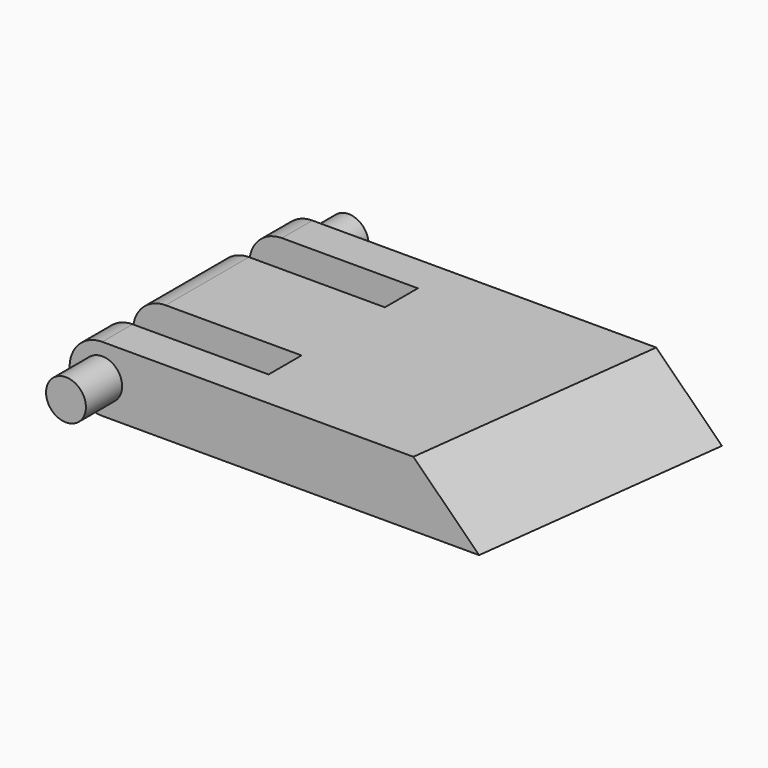
from build123d import *

# Parameters (mm, degrees)
F1_DEPTH  = 3.6
F2_SIZE2  = 3.59999
F2_SIZE   = 3.59999
F3_R      = 1.8
F4_R      = 1.79999
F5_R      = 1.8
F6_R      = 1.79999
F7_R      = 1.8
F8_R      = 1.79999
F9_R      = 1.1
F10_DEPTH = 2.5
F11_R     = 1.1
F12_DEPTH = 2.5


# Not quite as in the source:
# - a fillet or chamfer is up to 0.001 mm smaller than in the source, because OpenCascade refuses the exact size


with BuildPart() as f1:
    # F0 (on Top) → F1 (new body)
    with BuildSketch(Plane.XY):
        Polygon((24.4, 0), (0, 0), (0, -2.1), (9.3, -2.1), (9.3, -4.375), (0, -4.375), (0, -10.125), (9.3, -10.125), (9.3, -12.4), (0, -12.4), (0, -14.5), (22.6, -14.5), align=None)
    extrude(amount=F1_DEPTH)

    # F2 (size 3.6 and 3.6 in the source; OpenCascade refuses exactly that, so slightly less here)
    f2_edges = [f1.edges().sort_by_distance(p)[0] for p in [
        (23.5, -7.25, 3.6),
    ]]
    chamfer(f2_edges, length=F2_SIZE, length2=F2_SIZE2)

    # F3
    f3_edges = [f1.edges().sort_by_distance(p)[0] for p in [
        (0, -7.25, 3.6),
    ]]
    fillet(f3_edges, radius=F3_R)

    # F4 (radius 1.8 in the source; OpenCascade refuses exactly that, so slightly less here)
    f4_edges = [f1.edges().sort_by_distance(p)[0] for p in [
        (0, -7.25, 0),
    ]]
    fillet(f4_edges, radius=F4_R)

    # F5
    f5_edges = [f1.edges().sort_by_distance(p)[0] for p in [
        (0, -13.45, 3.6),
    ]]
    fillet(f5_edges, radius=F5_R)

    # F6 (radius 1.8 in the source; OpenCascade refuses exactly that, so slightly less here)
    f6_edges = [f1.edges().sort_by_distance(p)[0] for p in [
        (0, -13.45, 0),
    ]]
    fillet(f6_edges, radius=F6_R)

    # F7
    f7_edges = [f1.edges().sort_by_distance(p)[0] for p in [
        (0, -1.05, 3.6),
    ]]
    fillet(f7_edges, radius=F7_R)

    # F8 (radius 1.8 in the source; OpenCascade refuses exactly that, so slightly less here)
    f8_edges = [f1.edges().sort_by_distance(p)[0] for p in [
        (0, -1.05, 0),
    ]]
    fillet(f8_edges, radius=F8_R)

    # F9 (on face) → F10 (join)
    with BuildSketch(Plane.XZ.offset(14.5)):
        with Locations((1.8, 1.8)):
            Circle(F9_R)
    extrude(amount=F10_DEPTH)

    # F11 (on face) → F12 (join)
    with BuildSketch(Plane(origin=(0, 0, 0), x_dir=(-1, 0, 0), z_dir=(0, 1, 0))):
        with Locations((-1.8, 1.8)):
            Circle(F11_R)
    extrude(amount=F12_DEPTH)


solid = f1.part
